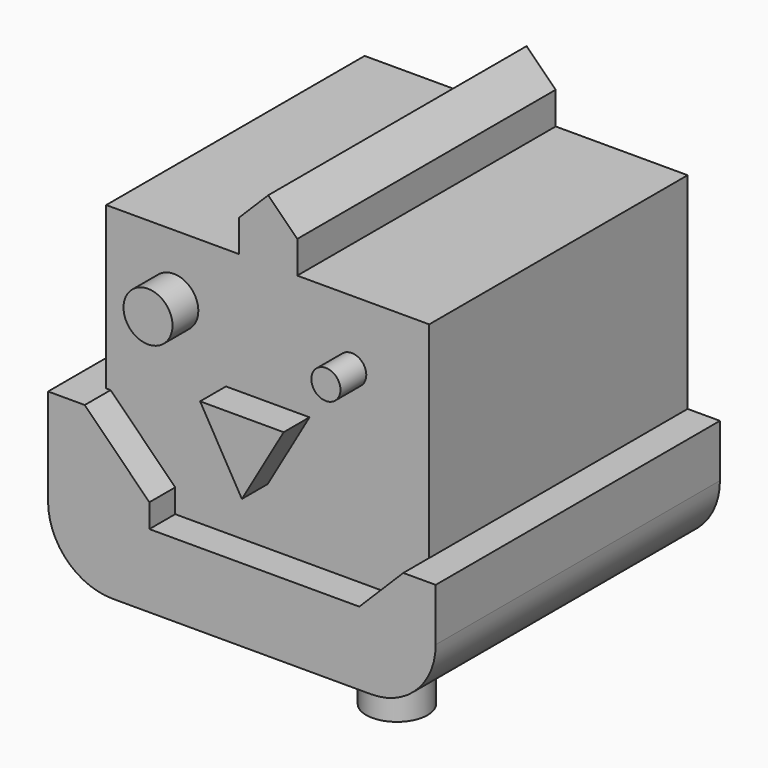
from build123d import *

# Parameters (mm, degrees)
F0_W         = 25.4
F0_H         = 25.4
F1_DEPTH     = 25.4
F2_W         = 5.424141106
F2_H         = 6.936683166
F2_W_2       = 5.0867797479
F2_H_2       = 3.4590791911
F3_DEPTH     = 2.54
F4_R         = 1.9260545118
F4_R_2       = 1.1454537096
F5_DEPTH     = 2.54
F7_DEPTH     = 2.54
F8_W         = 27.94
F8_H         = 9.2223960251
F9_DEPTH     = 2.54
F10_W        = 27.94
F10_H        = 12.7
F11_DEPTH    = 2.54
F12_T1_DEPTH = 15.6041495789
F12_T6_DEPTH = 15.6041495789
F13_W        = 4.5640636235
F13_H        = 25.4
F14_DEPTH    = 5.08
F15_T1_DEPTH = 38.4641495789
F16_R        = 5.08
F17_R        = 2.413
F18_DEPTH    = 10.16


# Not quite as in the source:
# - a fillet or chamfer that OpenCascade refuses, or shapes differently, is made with other operations: its cross-section is extruded or revolved along the edge and cut away or added


with BuildPart() as f1:
    # F0 (on Top) → F1 (new body)
    with BuildSketch(Plane.XY):
        Rectangle(F0_W, F0_H)
    extrude(amount=-F1_DEPTH)

    # F2 (on face) → F3 (join)
    with BuildSketch(Plane.XZ.offset(12.7)):
        Polygon((-12.7, -19.636683166), (-12.7, -25.4), (12.7, -25.4), (12.7, -19.636683166), (7.6132202521, -19.636683166), (-7.275858894, -19.636683166), align=None)
        with Locations((-9.987929447, -16.168341583)):
            Rectangle(F2_W, F2_H)
        with Locations((10.156610126, -17.9071435705)):
            Rectangle(F2_W_2, F2_H_2)
    extrude(amount=F3_DEPTH)

    # F4 (on face) → F5 (join)
    with BuildSketch(Plane.XZ.offset(12.7)):
        with Locations((-7.3823751882, -4.9585988745)):
            Circle(F4_R)
        with Locations((6.6054924391, -5.1089939661)):
            Circle(F4_R_2)
    extrude(amount=F5_DEPTH)

    # F6 (on face) → F7 (join)
    with BuildSketch(Plane.XZ.offset(12.7)):
        Polygon((3.2856935422, -9.4954269007), (-3.2856935422, -9.4954269007), (0, -15.1864150539), align=None)
    extrude(amount=F7_DEPTH)

    # F8 (on face) → F9 (join)
    with BuildSketch(Plane.YZ.offset(12.7)):
        with Locations((-1.27, -20.7888019875)):
            Rectangle(F8_W, F8_H)
    extrude(amount=F9_DEPTH)

    # F10 (on face) → F11 (join)
    with BuildSketch(Plane(origin=(-12.7, 0, 0), x_dir=(0, -1, 0), z_dir=(-1, 0, 0))):
        with Locations((1.27, -19.05)):
            Rectangle(F10_W, F10_H)
    extrude(amount=F11_DEPTH)

    # F12: chamfer of 5.08 on 2 edges, made by hand

    # F12_s2 → F12_t1 (cut)
    with BuildSketch(Plane.XZ.offset(12.7)):
        Polygon((-7.275858894, -17.78), (-12.355858894, -12.7), (-7.275858894, -12.7), align=None)
    extrude(amount=F12_T1_DEPTH, mode=Mode.SUBTRACT)


with BuildPart() as f12_tool4:
    # F12_s5 → F12_t6 (new body)
    with BuildSketch(Plane.XZ.offset(12.7)):
        Polygon((7.6132202521, -21.2576039749), (12.6932202521, -16.1776039749), (7.6132202521, -16.1776039749), align=None)
    extrude(amount=F12_T6_DEPTH)

    split(bisect_by=Plane.XY.offset(-19.636683166), keep=Keep.TOP)


with BuildPart() as f1_1:
    add(f1.part)

    # F12_t3: cut F12_tool4
    add(f12_tool4.part, mode=Mode.SUBTRACT)

    # F13 (on face) → F14 (join)
    with BuildSketch(Plane.XY):
        with Locations((0.04063081, 0)):
            Rectangle(F13_W, F13_H)
    extrude(amount=F14_DEPTH)

    # F15: chamfer of 2.54 on 2 edges, made by hand

    # F15_s2 → F15_t1 (cut)
    with BuildSketch(Plane.XZ.offset(-19.2320747894)):
        Polygon((2.3226626217, 2.54), (-0.2173373783, 5.08), (2.3226626217, 5.08), align=None)
        Polygon((-2.2414010018, 2.54), (0.2985989982, 5.08), (-2.2414010018, 5.08), align=None)
    extrude(amount=F15_T1_DEPTH, mode=Mode.SUBTRACT)

    # F16
    f16_edges = [f1_1.edges().sort_by_distance(p)[0] for p in [
        (15.24, -1.27, -25.4),
        (-15.24, -1.27, -25.4),
    ]]
    fillet(f16_edges, radius=F16_R)

    # F17 (on face) → F18 (join)
    with BuildSketch(Plane(origin=(0, 0, -25.4), x_dir=(1, 0, 0), z_dir=(0, 0, -1))):
        Circle(F17_R)
    extrude(amount=F18_DEPTH)


solid = f1_1.part
